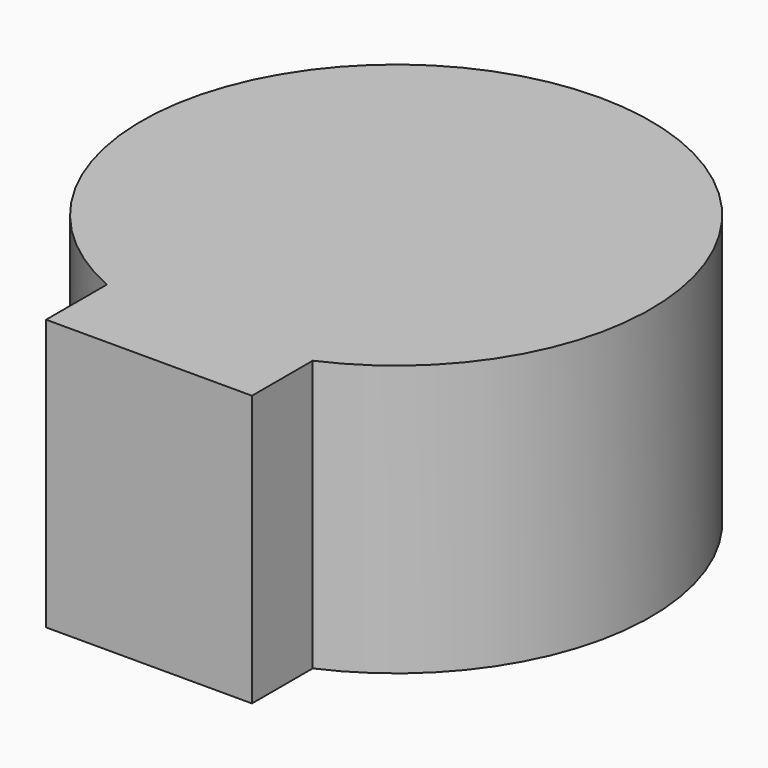
from build123d import *

# Parameters (mm, degrees)
F0_R     = 23.5
F1_DEPTH = 25
F2_W     = 19
F2_H     = 10
F3_DEPTH = 25
F5_DEPTH = 20


# Not quite as in the source:
# - a feature names something its author has since deleted; it is built from what else it names


with BuildPart() as f1:
    # F0 (on Top) → F1 (new body)
    with BuildSketch(Plane.XY):
        Circle(F0_R)
    extrude(amount=F1_DEPTH)

    # F2 (on face) → F3 (join)
    with BuildSketch(Plane.XY.offset(25)):
        with Locations((0, -23.5)):
            Rectangle(F2_W, F2_H)
    extrude(amount=-F3_DEPTH)

    # F4 (on Top) → F5 (cut)
    with BuildSketch(Plane.XY):
        with BuildLine():
            Line((-0.1196338324, -26.5), (-0.094803203, -20.9997860073))
            ThreePointArc((-0.094803203, -20.9997860073), (-3.6604096567, -20.6785251202), (-7.1196338324, -19.7562854325))
            Line((-7.1196338324, -19.7562854325), (-7.1196338324, -26.5))
            Line((-7.1196338324, -26.5), (-0.1196338324, -26.5))
        make_face()
        with BuildLine():
            ThreePointArc((6.8803661676, -19.8408810641), (3.4419080977, -20.7160147868), (-0.094803203, -20.9997860073))
            Line((-0.094803203, -20.9997860073), (-0.1196338324, -26.5))
            Line((-0.1196338324, -26.5), (6.8803661676, -26.5))
            Line((6.8803661676, -26.5), (6.8803661676, -19.8408810641))
        make_face()
        with BuildLine():
            ThreePointArc((-7.1196338324, -19.7562854325), (-3.6604096567, -20.6785251202), (-0.094803203, -20.9997860073))
            ThreePointArc((-0.094803203, -20.9997860073), (3.4419080977, -20.7160147868), (6.8803661676, -19.8408810641))
            ThreePointArc((6.8803661676, -19.8408810641), (17.1097587581, -12.1760484247), (21, 0))
            ThreePointArc((21, 0), (-12.0724415409, 17.1830193866), (-7.1196338324, -19.7562854325))
        make_face()
    extrude(amount=F5_DEPTH, mode=Mode.SUBTRACT)


solid = f1.part
